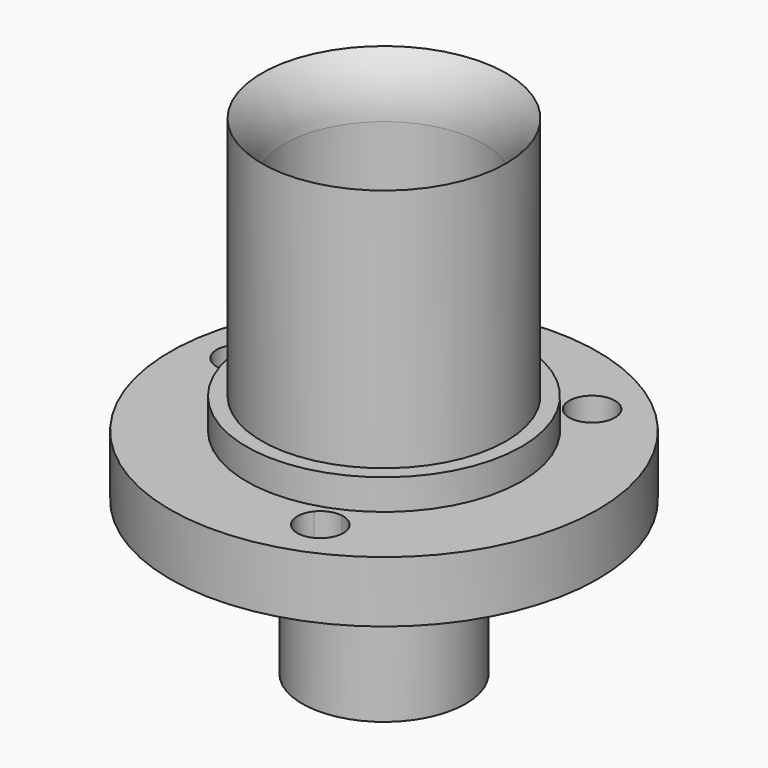
from build123d import *

# Parameters (mm, degrees)
F0_R      = 14
F0_R_2    = 3.15
F1_DEPTH  = 4
F2_R      = 9
F3_DEPTH  = 6
F4_R      = 8
F5_DEPTH  = 22
F6_R      = 6.5
F7_DEPTH  = 25
F10_DEPTH = 2
F11_DEPTH = 25
F9_R      = 5.35
F9_R_2    = 3.15
F12_DEPTH = 10


# Not quite as in the source:
# - a fillet or chamfer that OpenCascade refuses, or shapes differently, is made with other operations: its cross-section is extruded or revolved along the edge and cut away or added


with BuildPart() as f1:
    # F0 (on Top) → F1 (new body)
    with BuildSketch(Plane.XY):
        Circle(F0_R)
        Circle(F0_R_2, mode=Mode.SUBTRACT)
    extrude(amount=F1_DEPTH)

    # F2 (on Top) → F3 (join)
    with BuildSketch(Plane.XY):
        Circle(F2_R)
    extrude(amount=F3_DEPTH)

    # F4 (on Top) → F5 (join)
    with BuildSketch(Plane.XY):
        Circle(F4_R)
    extrude(amount=F5_DEPTH)

    # F6 (on Top) → F7 (cut)
    with BuildSketch(Plane.XY):
        Circle(F6_R)
    extrude(amount=F7_DEPTH, mode=Mode.SUBTRACT)

    # F0 (on Top) → F10 (join)
    with BuildSketch(Plane.XY):
        Circle(F0_R)
        Circle(F0_R_2, mode=Mode.SUBTRACT)
    extrude(amount=F10_DEPTH)

    # F8 (on Top) → F11 (cut)
    with BuildSketch(Plane.XY):
        with BuildLine():
            Line((3.9571776785, -10.1563155141), (2.7867408683, -9.2181909629))
            ThreePointArc((2.7867408683, -9.2181909629), (3.460013327, -11.5715284336), (5.4571776785, -10.1563155141))
            ThreePointArc((5.4571776785, -10.1563155141), (5.0953410965, -9.1792873497), (4.1843989666, -8.6736252274))
            Line((4.1843989666, -8.6736252274), (3.9571776785, -10.1563155141))
        make_face()
        with BuildLine():
            ThreePointArc((4.1843989666, -8.6736252274), (3.4126119429, -8.7586574158), (2.7867408683, -9.2181909629))
            Line((2.7867408683, -9.2181909629), (3.9571776785, -10.1563155141))
            Line((3.9571776785, -10.1563155141), (4.1843989666, -8.6736252274))
        make_face()
        with BuildLine():
            Line((-9.6037792731, 0.7130168091), (-10.7742160833, 1.6511413602))
            Line((-10.7742160833, 1.6511413602), (-9.376557985, 2.1957070958))
            ThreePointArc((-9.376557985, 2.1957070958), (-12.2569063699, 1.8783626483), (-9.6037792731, 0.7130168091))
        make_face()
        with BuildLine():
            Line((-9.376557985, 2.1957070958), (-10.7742160833, 1.6511413602))
            Line((-10.7742160833, 1.6511413602), (-9.6037792731, 0.7130168091))
            ThreePointArc((-9.6037792731, 0.7130168091), (-9.3590031637, 1.1539770087), (-9.2742160833, 1.6511413602))
            ThreePointArc((-9.2742160833, 1.6511413602), (-9.3000235674, 1.9281908617), (-9.376557985, 2.1957070958))
        make_face()
        with BuildLine():
            ThreePointArc((8.3170384048, 8.5051741539), (6.5399889033, 9.9793666697), (5.4193803065, 7.9606084183))
            Line((5.4193803065, 7.9606084183), (6.8170384048, 8.5051741539))
            Line((6.8170384048, 8.5051741539), (6.5898171167, 7.0224838672))
            ThreePointArc((6.5898171167, 7.0224838672), (7.7940665691, 7.3670107359), (8.3170384048, 8.5051741539))
        make_face()
        with BuildLine():
            Line((6.8170384048, 8.5051741539), (5.4193803065, 7.9606084183))
            ThreePointArc((5.4193803065, 7.9606084183), (5.8789138537, 7.3347373437), (6.5898171167, 7.0224838672))
            Line((6.5898171167, 7.0224838672), (6.8170384048, 8.5051741539))
        make_face()
    extrude(amount=F11_DEPTH, mode=Mode.SUBTRACT)

    # F9 (on Top) → F12 (join)
    with BuildSketch(Plane.XY):
        Circle(F9_R)
        Circle(F9_R_2, mode=Mode.SUBTRACT)
    extrude(amount=-F12_DEPTH)

    # F13: fillet of radius 5 on 1 edges, made by hand

    # F13_s1 → F13_t2 (revolve, cut)
    with BuildSketch(Plane.XZ):
        with BuildLine():
            ThreePointArc((8, 22), (6.8902277714, 20.3657774588), (6.5, 18.4292857857))
            Line((6.5, 18.4292857857), (6.5, 22))
            Line((6.5, 22), (8, 22))
        make_face()
    revolve(axis=Axis((0, 0, 22), (0, 0, -1)), mode=Mode.SUBTRACT)


solid = f1.part
